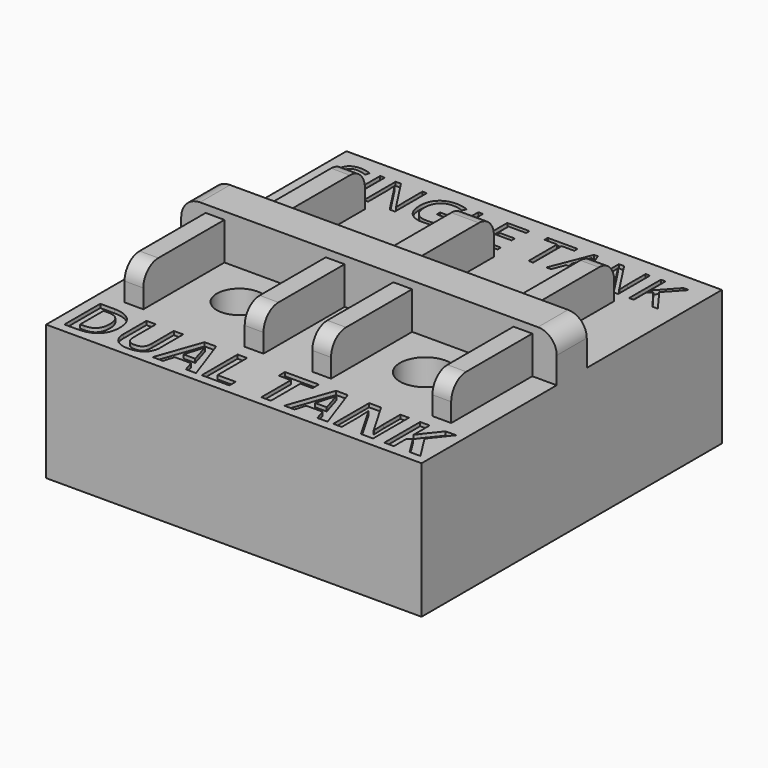
from build123d import *

# Parameters (mm, degrees)
F0_W          = 100
F0_H          = 100
F0_R          = 6
F1_DEPTH      = 36
F2_W          = 100
F2_H          = 10
F3_DEPTH      = 12
F4_W          = 5
F4_H          = 27
F5_DEPTH      = 10
F6_W          = 5
F6_H          = 27
F6_W_2        = 7.364
F7_DEPTH      = 10
F8_R          = 6.75
F9_DEPTH      = 30.58
F10_R         = 4.65
F11_DEPTH     = 15
F12_TEXT_SIZE = 16.7298027211
F13_DEPTH     = 1
F15_R         = 5
F14_TEXT_SIZE = 14.8488174833
F16_DEPTH     = 1


# Not quite as in the source:
# - Text() gives the source's letters only with a copy of the font that has no kerning and outlines rounded to 1/6400 em; it was checked with that copy


with BuildPart() as f1:
    # F0 (on Top) → F1 (new body)
    with BuildSketch(Plane.XY):
        Rectangle(F0_W, F0_H)
        with Locations((-25, -16.9)):
            Circle(F0_R, mode=Mode.SUBTRACT)
        with Locations((-18, 16.9)):
            Circle(F0_R, mode=Mode.SUBTRACT)
        with Locations((18, 16.9)):
            Circle(F0_R, mode=Mode.SUBTRACT)
    extrude(amount=F1_DEPTH)

    # F2 (on face) → F3 (join)
    with BuildSketch(Plane.XY.offset(36)):
        Rectangle(F2_W, F2_H)
    extrude(amount=F3_DEPTH)

    # F4 (on face) → F5 (join)
    with BuildSketch(Plane.XY.offset(36)):
        with Locations((41, -18.5)):
            Rectangle(F4_W, F4_H)
        with Locations((9, -18.5)):
            Rectangle(F4_W, F4_H)
        with Locations((-9, -18.5)):
            Rectangle(F4_W, F4_H)
        with Locations((-41, -18.5)):
            Rectangle(F4_W, F4_H)
    extrude(amount=F5_DEPTH)

    # F6 (on face) → F7 (join)
    with BuildSketch(Plane.XY.offset(36)):
        with Locations((-33.1818176806, 18.5)):
            Rectangle(F6_W, F6_H)
        with Locations((0.0001823194, 18.5)):
            Rectangle(F6_W_2, F6_H)
        with Locations((33.1821823194, 18.5)):
            Rectangle(F6_W, F6_H)
    extrude(amount=F7_DEPTH)

    # F8 (on face) → F9 (cut)
    with BuildSketch(Plane.XY.offset(36)):
        with Locations((25, -17.5)):
            Circle(F8_R)
    extrude(amount=-F9_DEPTH, mode=Mode.SUBTRACT)

    # F10 (on face) → F11 (join)
    with BuildSketch(Plane.XY.offset(5.42)):
        with Locations((25, -17.5)):
            Circle(F10_R)
    extrude(amount=F11_DEPTH)

    # F12 (on face) → F13 (cut)
    with BuildSketch(Plane.XY.offset(36)):
        with Locations((-48.5584978014, -47.5885607302)):
            Text('DUAL TANK', F12_TEXT_SIZE, font='Open Sans', font_style=FontStyle.BOLD, text_align=(TextAlign.LEFT, TextAlign.BOTTOM))
    extrude(amount=-F13_DEPTH, mode=Mode.SUBTRACT)

    # F15
    f15_edges = [f1.edges().sort_by_distance(p)[0] for p in [
        (-50, 0, 48),
        (50, 0, 48),
        (41, -32, 46),
        (9, -32, 46),
        (-9, -32, 46),
        (-41, -32, 46),
        (-33.181818, 32, 46),
        (0.000182, 32, 46),
        (33.182182, 32, 46),
    ]]
    fillet(f15_edges, radius=F15_R)

    # F14 (on face) → F16 (cut)
    with BuildSketch(Plane.XY.offset(36)):
        with Locations((-47.1668515107, 35.073598968)):
            Text('SINGLE TANK', F14_TEXT_SIZE, font='Open Sans', text_align=(TextAlign.LEFT, TextAlign.BOTTOM))
    extrude(amount=-F16_DEPTH, mode=Mode.SUBTRACT)


solid = f1.part
